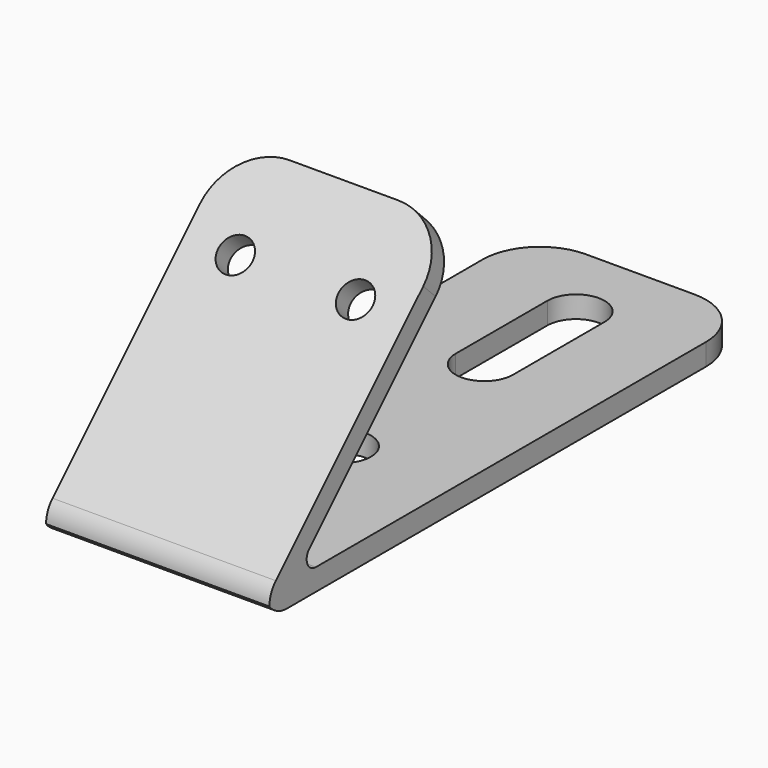
from build123d import *

# Parameters (mm, degrees)
F1_DEPTH    = 247.65
F2_R        = 127
F3_R        = 25.4
F4_R        = 60.96
F5_T1_DEPTH = 736.9542394832
F6_R        = 38.1
F7_DEPTH    = 132.08
F8_R        = 63.5
F9_DEPTH    = 111.76


# Not quite as in the source:
# - a fillet or chamfer that OpenCascade refuses, or shapes differently, is made with other operations: its cross-section is extruded or revolved along the edge and cut away or added


with BuildPart() as f1:
    # F0 (on Right) → F1 (new body, symmetric)
    with BuildSketch(Plane.YZ):
        Polygon((-67.451213715, 0), (0, 0), (1270, 0), (1270, 48.26), (0, 48.26), (483.1377793135, 531.3977793135), (449.0128060535, 565.5227525736), (0, 116.5099465201), (-67.451213715, 49.0587328052), align=None)
    extrude(amount=F1_DEPTH, both=True)

    # F2
    f2_edges = [f1.edges().sort_by_distance(p)[0] for p in [
        (247.65, 466.075293, 548.460266),
        (-247.65, 466.075293, 548.460266),
        (247.65, 1270, 24.13),
        (-247.65, 1270, 24.13),
    ]]
    fillet(f2_edges, radius=F2_R)

    # F3
    f3_edges = [f1.edges().sort_by_distance(p)[0] for p in [
        (0, 0, 48.26),
    ]]
    fillet(f3_edges, radius=F3_R)

    # F4
    f4_edges = [f1.edges().sort_by_distance(p)[0] for p in [
        (0, -67.451214, 49.058733),
    ]]
    fillet(f4_edges, radius=F4_R)

    # F5: fillet of radius 60.96 on 1 edges, made by hand

    # F5_s2 → F5_t1 (cut)
    with BuildSketch(Plane.YZ.offset(-368.4771197416)):
        with BuildLine():
            ThreePointArc((-67.451213715, 23.8082740429), (-46.0587435131, 6.2750349075), (-19.1203658183, 0))
            Line((-19.1203658183, 0), (-67.451213715, 0))
            Line((-67.451213715, 0), (-67.451213715, 23.8082740429))
        make_face()
    extrude(amount=F5_T1_DEPTH, mode=Mode.SUBTRACT)

    # F6 (on face) → F7 (cut)
    with BuildSketch(Plane(origin=(0, -58.2549732601, 58.2549732601), x_dir=(1, 0, 0), z_dir=(0, -0.7071067812, 0.7071067812))):
        with Locations((-133.35, 526.8849732601)):
            Circle(F6_R)
        with Locations((133.35, 526.8849732601)):
            Circle(F6_R)
    extrude(amount=-F7_DEPTH, mode=Mode.SUBTRACT)

    # F8 (on Top) → F9 (cut)
    with BuildSketch(Plane.XY):
        with Locations((0, 444.5)):
            Circle(F8_R)
        with BuildLine():
            Line((-63.5, 838.2), (63.5, 838.2))
            ThreePointArc((63.5, 838.2), (0, 901.7), (-63.5, 838.2))
        make_face()
        with BuildLine():
            ThreePointArc((-63.5, 838.2), (0, 774.7), (63.5, 838.2))
            Line((63.5, 838.2), (-63.5, 838.2))
        make_face()
        with BuildLine():
            ThreePointArc((-63.5, 838.2), (0, 901.7), (63.5, 838.2))
            Line((63.5, 838.2), (63.5, 1092.2))
            ThreePointArc((63.5, 1092.2), (0, 1028.7), (-63.5, 1092.2))
            Line((-63.5, 1092.2), (-63.5, 838.2))
        make_face()
        with BuildLine():
            Line((-63.5, 1092.2), (63.5, 1092.2))
            ThreePointArc((63.5, 1092.2), (0, 1155.7), (-63.5, 1092.2))
        make_face()
        with BuildLine():
            ThreePointArc((-63.5, 1092.2), (0, 1028.7), (63.5, 1092.2))
            Line((63.5, 1092.2), (-63.5, 1092.2))
        make_face()
    extrude(amount=F9_DEPTH, mode=Mode.SUBTRACT)


solid = f1.part
